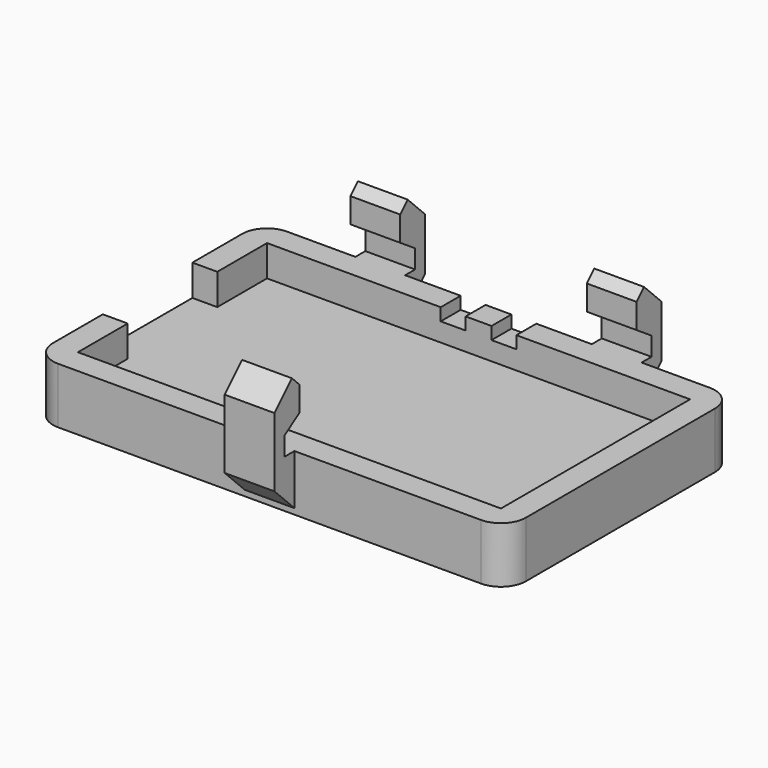
from build123d import *

# Parameters (mm, degrees)
F0_W          = 38
F0_H          = 23
F1_DEPTH      = 4.5
F2_T          = -2
F3_W          = 9
F3_H          = 2.5
F4_DEPTH      = 2
F5_W          = 2
F5_H          = 1
F6_DEPTH      = 2
F7_W          = 4
F7_H          = 4
F7_H_2        = 4.2236842105
F8_DEPTH      = 2
F9_DEPTH      = 0.5
F10_W         = 4
F10_H         = 4
F10_H_2       = 5.5396806626
F11_DEPTH     = 2
F12_DEPTH     = 0.5
F13_SIZE2     = 1
F13_SIZE      = 1
F14_T1_DEPTH  = 14.2867319519
F14_T3_DEPTH  = 14.2867319519
F14_T5_DEPTH  = 14.2867319519
F14_T10_DEPTH = 14.2867319519
F14_T15_DEPTH = 14.2867319519
F14_T20_DEPTH = 14.2867319519
F15_R         = 2
F10_H_3       = 1.5
F16_DEPTH     = 1
F7_H_3        = 1.5
F17_DEPTH     = 1
F18_SIZE2     = 0.99999
F18_SIZE      = 1.49999
F19_SIZE2     = 1.49999
F19_SIZE      = 0.99999
F20_SIZE2     = 0.99999
F20_SIZE      = 1.49999


# Not quite as in the source:
# - a fillet or chamfer that OpenCascade refuses, or shapes differently, is made with other operations: its cross-section is extruded or revolved along the edge and cut away or added
# - a fillet or chamfer is up to 0.001 mm smaller than in the source, because OpenCascade refuses the exact size


with BuildPart() as f1:
    # F0 (on Top) → F1 (new body)
    with BuildSketch(Plane.XY):
        Rectangle(F0_W, F0_H)
    extrude(amount=F1_DEPTH)

    # F2
    f2_openings = [f1.faces().sort_by_distance(p)[0] for p in [
        (0, 0, 4.5),
    ]]
    offset(amount=F2_T, openings=f2_openings)

    # F3 (on face) → F4 (cut, through all)
    with BuildSketch(Plane(origin=(-19, 0, 0), x_dir=(0, -1, 0), z_dir=(-1, 0, 0))):
        with Locations((0, 3.25)):
            Rectangle(F3_W, F3_H)
    extrude(amount=-F4_DEPTH, mode=Mode.SUBTRACT)

    # F5 (on face) → F6 (cut, through all)
    with BuildSketch(Plane(origin=(0, 11.5, 0), x_dir=(-1, 0, 0), z_dir=(0, 1, 0))):
        with Locations((-2.0402920675, 4)):
            Rectangle(F5_W, F5_H)
        with Locations((2.0402920675, 4)):
            Rectangle(F5_W, F5_H)
    extrude(amount=-F6_DEPTH, mode=Mode.SUBTRACT)

    # F7 (on face) → F8 (join)
    with BuildSketch(Plane(origin=(0, 11.5, 0), x_dir=(-1, 0, 0), z_dir=(0, 1, 0))):
        with Locations((-9.5, 8)):
            Rectangle(F7_W, F7_H)
        with Locations((-9.5, 3.8881578947)):
            Rectangle(F7_W, F7_H_2)
        with Locations((9.5, 8)):
            Rectangle(F7_W, F7_H)
        with Locations((9.5, 3.8881578947)):
            Rectangle(F7_W, F7_H_2)
    extrude(amount=F8_DEPTH)

    # F7 (on face) → F9 (join)
    with BuildSketch(Plane(origin=(0, 11.5, 0), x_dir=(-1, 0, 0), z_dir=(0, 1, 0))):
        with Locations((-9.5, 8)):
            Rectangle(F7_W, F7_H)
        with Locations((9.5, 8)):
            Rectangle(F7_W, F7_H)
    extrude(amount=-F9_DEPTH)

    # F10 (on face) → F11 (join)
    with BuildSketch(Plane.XZ.offset(11.5)):
        with Locations((0, 8)):
            Rectangle(F10_W, F10_H)
        with Locations((0, 3.2301596687)):
            Rectangle(F10_W, F10_H_2)
    extrude(amount=F11_DEPTH)

    # F10 (on face) → F12 (join)
    with BuildSketch(Plane.XZ.offset(11.5)):
        with Locations((0, 8)):
            Rectangle(F10_W, F10_H)
    extrude(amount=-F12_DEPTH)

    # F13
    f13_edges = [f1.edges().sort_by_distance(p)[0] for p in [
        (0, -11, 10),
        (-9.5, 11, 10),
        (9.5, 11, 10),
    ]]
    chamfer(f13_edges, length=F13_SIZE, length2=F13_SIZE2)

    # F14: chamfer of 2 on 6 edges, made by hand

    # F14_s2 → F14_t1 (cut)
    with BuildSketch(Plane.YZ.offset(2.3566340241)):
        Polygon((11.5, 10), (13.5, 8), (13.5, 10), align=None)
    extrude(amount=F14_T1_DEPTH, mode=Mode.SUBTRACT)

    # F14_s4 → F14_t3 (cut)
    with BuildSketch(Plane.YZ.offset(-16.6433659759)):
        Polygon((11.5, 10), (13.5, 8), (13.5, 10), align=None)
    extrude(amount=F14_T3_DEPTH, mode=Mode.SUBTRACT)

    # F14_s6 → F14_t5 (cut)
    with BuildSketch(Plane.YZ.offset(-7.1433659759)):
        Polygon((-11.5, 10), (-13.5, 8), (-13.5, 10), align=None)
    extrude(amount=F14_T5_DEPTH, mode=Mode.SUBTRACT)


with BuildPart() as f14_tool8:
    # F14_s9 → F14_t10 (new body)
    with BuildSketch(Plane.YZ.offset(-2.3566340241)):
        Polygon((11.5, 1.7763157895), (13.5, 3.7763157895), (13.5, 1.7763157895), align=None)
    extrude(amount=-F14_T10_DEPTH)

    split(bisect_by=Plane.XZ.offset(-11.5), keep=Keep.BOTTOM)


with BuildPart() as f1_1:
    add(f1.part)

    # F14_t7: cut F14_tool8
    add(f14_tool8.part, mode=Mode.SUBTRACT)


with BuildPart() as f14_tool13:
    # F14_s14 → F14_t15 (new body)
    with BuildSketch(Plane.YZ.offset(16.6433659759)):
        Polygon((13.5, 3.7763157895), (11.5, 1.7763157895), (13.5, 1.7763157895), align=None)
    extrude(amount=-F14_T15_DEPTH)

    split(bisect_by=Plane.XZ.offset(-11.5), keep=Keep.BOTTOM)


with BuildPart() as f1_2:
    add(f1_1.part)

    # F14_t12: cut F14_tool13
    add(f14_tool13.part, mode=Mode.SUBTRACT)


with BuildPart() as f14_tool18:
    # F14_s19 → F14_t20 (new body)
    with BuildSketch(Plane.YZ.offset(-7.1433659759)):
        Polygon((-11.5, 0.4603193374), (-13.5, 2.4603193374), (-13.5, 0.4603193374), align=None)
    extrude(amount=F14_T20_DEPTH)

    split(bisect_by=Plane.XZ.offset(11.5), keep=Keep.TOP)


with BuildPart() as f1_3:
    add(f1_2.part)

    # F14_t17: cut F14_tool18
    add(f14_tool18.part, mode=Mode.SUBTRACT)

    # F15
    f15_edges = [f1_3.edges().sort_by_distance(p)[0] for p in [
        (19, -11.5, 2.25),
        (19, 11.5, 2.25),
        (-19, 11.5, 2.25),
        (-19, -11.5, 2.25),
    ]]
    fillet(f15_edges, radius=F15_R)

    # F10 (on face) → F16 (cut)
    with BuildSketch(Plane.XZ.offset(11.5)):
        with Locations((0, 5.25)):
            Rectangle(F10_W, F10_H_3)
    extrude(amount=F16_DEPTH, mode=Mode.SUBTRACT)

    # F7 (on face) → F17 (cut)
    with BuildSketch(Plane(origin=(0, 11.5, 0), x_dir=(-1, 0, 0), z_dir=(0, 1, 0))):
        with Locations((9.5, 5.25)):
            Rectangle(F7_W, F7_H_3)
        with Locations((-9.5, 5.25)):
            Rectangle(F7_W, F7_H_3)
    extrude(amount=F17_DEPTH, mode=Mode.SUBTRACT)

    # F18 (size 1.5 and 1 in the source; OpenCascade refuses exactly that, so slightly less here)
    f18_edges = [f1_3.edges().sort_by_distance(p)[0] for p in [
        (0, -11, 6),
    ]]
    f18_side = f1_3.faces().sort_by_distance((0, -11.75, 6))[0]
    chamfer(f18_edges, length=F18_SIZE, length2=F18_SIZE2, reference=f18_side)

    # F19 (size 1 and 1.5 in the source; OpenCascade refuses exactly that, so slightly less here)
    f19_edges = [f1_3.edges().sort_by_distance(p)[0] for p in [
        (-9.5, 11, 6),
    ]]
    f19_side = f1_3.faces().sort_by_distance((-9.5, 11, 7.5))[0]
    chamfer(f19_edges, length=F19_SIZE, length2=F19_SIZE2, reference=f19_side)

    # F20 (size 1.5 and 1 in the source; OpenCascade refuses exactly that, so slightly less here)
    f20_edges = [f1_3.edges().sort_by_distance(p)[0] for p in [
        (9.5, 11, 6),
    ]]
    f20_side = f1_3.faces().sort_by_distance((9.5, 11.75, 6))[0]
    chamfer(f20_edges, length=F20_SIZE, length2=F20_SIZE2, reference=f20_side)


solid = f1_3.part
